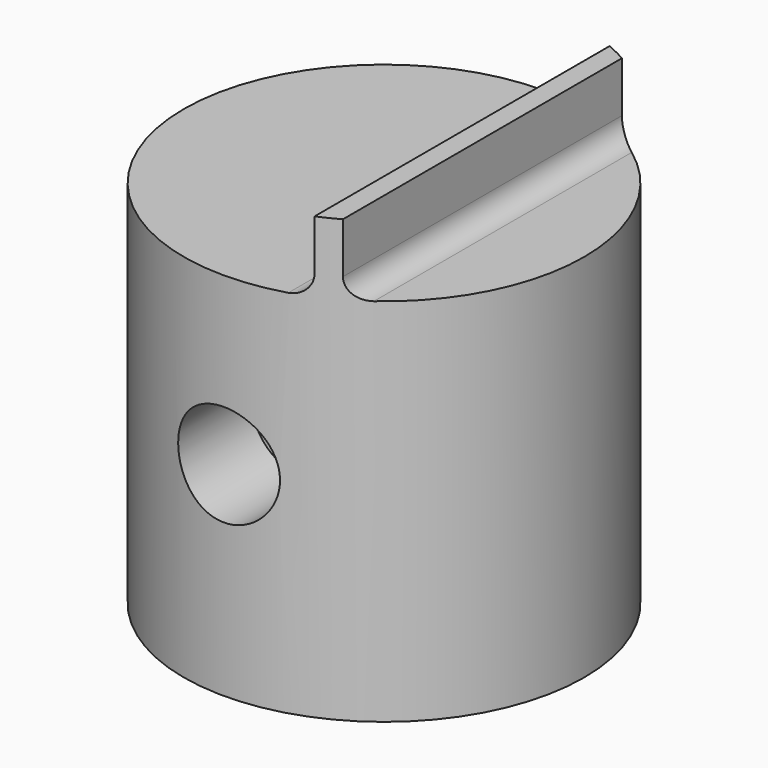
from build123d import *

# Parameters (mm, degrees)
F0_W      = 11.8
F0_H      = 21.82
F3_W      = 1.2
F3_H      = 40
F4_DEPTH  = 26
F5_R      = 11.8
F6_DEPTH  = 30
F2_W      = 11.2
F2_H      = 8
F9_W      = 21
F9_H      = 12
F10_DEPTH = 20
F11_R     = 5.99999
F13_R     = 1.2
F14_R     = 3
F15_DEPTH = 12.5


# Not quite as in the source:
# - a fillet or chamfer is up to 0.001 mm smaller than in the source, because OpenCascade refuses the exact size


with BuildPart() as f1:
    # F0 (on Front) → F1 (revolve)
    with BuildSketch(Plane.XZ):
        with Locations((5.9, 10.91)):
            Rectangle(F0_W, F0_H)
    revolve(axis=Axis((0, 0, 10.91), (0, 0, 1)))


with BuildPart() as f4:
    # F3 (on Top) → F4 (new body)
    with BuildSketch(Plane.XY):
        with Locations((5.2, 0)):
            Rectangle(F3_W, F3_H)
    extrude(amount=F4_DEPTH)


with BuildPart() as f6_tool:
    # F5 (on Top) → F6 (new body)
    with BuildSketch(Plane.XY):
        Circle(F5_R)
    extrude(amount=F6_DEPTH)


with BuildPart() as f1_1:
    add(f1.part)

    # F6: intersect by f6_tool
    add(f6_tool.part, mode=Mode.INTERSECT)


with BuildPart() as f4_1:
    add(f4.part)

    # F6: intersect by f6_tool
    add(f6_tool.part, mode=Mode.INTERSECT)

    # F7: union F1
    add(f1_1.part)

    # F2 (on Front) → F8 (revolve, cut)
    with BuildSketch(Plane.XZ):
        with Locations((5.6, 4)):
            Rectangle(F2_W, F2_H)
    revolve(axis=Axis((0, 0, 4), (0, 0, 1)), mode=Mode.SUBTRACT)


with BuildPart() as f10:
    # F9 (on Top) → F10 (new body)
    with BuildSketch(Plane.XY):
        Rectangle(F9_W, F9_H)
    extrude(amount=F10_DEPTH)

    # F11 (radius 6 in the source; OpenCascade refuses exactly that, so slightly less here)
    f11_edges = [f10.edges().sort_by_distance(p)[0] for p in [
        (-10.5, -6, 10),
        (10.5, -6, 10),
        (-10.5, 6, 10),
        (10.5, 6, 10),
    ]]
    fillet(f11_edges, radius=F11_R)


with BuildPart() as f4_2:
    add(f4_1.part)

    # F12: cut F10
    add(f10.part, mode=Mode.SUBTRACT)

    # F13
    f13_edges = [f4_2.edges().sort_by_distance(p)[0] for p in [
        (4.6, 0, 21.82),
        (5.8, 0, 21.82),
    ]]
    fillet(f13_edges, radius=F13_R)

    # F14 (on Front) → F15 (cut, symmetric)
    with BuildSketch(Plane.XZ):
        with Locations((0, 12)):
            Circle(F14_R)
    extrude(amount=F15_DEPTH, both=True, mode=Mode.SUBTRACT)


solid = f4_2.part
